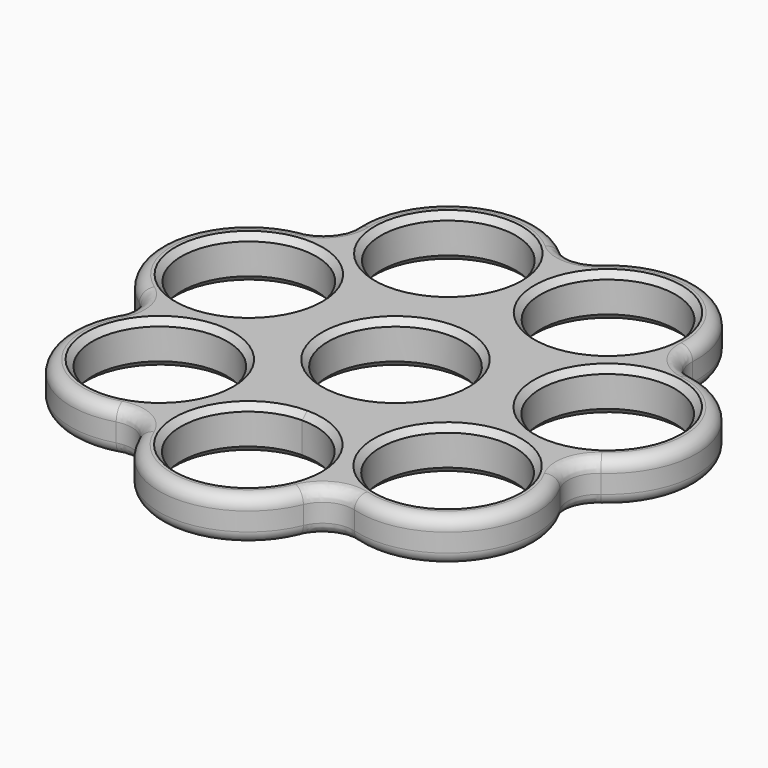
from build123d import *

# Parameters (mm, degrees)
F1_DEPTH = 7
F3_COUNT = 7
F5_R     = 11
F6_DEPTH = 7.001
F7_R     = 5
F8_R     = 2
F9_SIZE  = 1


# Not quite as in the source:
# - a feature names something its author has since deleted; it is built from what else it names


with BuildPart() as f1:
    # F0 (on Top) → F1 (new body)
    with BuildSketch(Plane.XY):
        with BuildLine():
            ThreePointArc((-14.5, 0), (0, -14.5), (14.5, 0))
            ThreePointArc((14.5, 0), (0, 14.5), (-14.5, 0))
        make_face()
        with BuildLine():
            Line((14.5, -30), (14.5, 0))
            ThreePointArc((14.5, 0), (0, -14.5), (-14.5, 0))
            Line((-14.5, 0), (-14.5, -30))
            ThreePointArc((-14.5, -30), (0, -15.5), (14.5, -30))
        make_face()
        with BuildLine():
            ThreePointArc((-14.5, -30), (0, -44.5), (14.5, -30))
            ThreePointArc((14.5, -30), (0, -15.5), (-14.5, -30))
        make_face()
    extrude(amount=F1_DEPTH)


with BuildPart() as f3_1:
    # F3: instance of F1
    add(f1.part.rotate(Axis((0, 0, 13.2415927947), (0, 0, 1)), 1 * 360 / F3_COUNT))


with BuildPart() as f3_2:
    # F3: instance of F1
    add(f1.part.rotate(Axis((0, 0, 13.2415927947), (0, 0, 1)), 2 * 360 / F3_COUNT))


with BuildPart() as f3_3:
    # F3: instance of F1
    add(f1.part.rotate(Axis((0, 0, 13.2415927947), (0, 0, 1)), 3 * 360 / F3_COUNT))


with BuildPart() as f3_4:
    # F3: instance of F1
    add(f1.part.rotate(Axis((0, 0, 13.2415927947), (0, 0, 1)), 4 * 360 / F3_COUNT))


with BuildPart() as f3_5:
    # F3: instance of F1
    add(f1.part.rotate(Axis((0, 0, 13.2415927947), (0, 0, 1)), 5 * 360 / F3_COUNT))


with BuildPart() as f3_6:
    # F3: instance of F1
    add(f1.part.rotate(Axis((0, 0, 13.2415927947), (0, 0, 1)), 6 * 360 / F3_COUNT))


with BuildPart() as f3_5_1:
    add(f3_5.part)

    # F4: union F3_6, F1, F3_1, F3_2, F3_3, F3_4
    add(f3_6.part)
    add(f1.part)
    add(f3_1.part)
    add(f3_2.part)
    add(f3_3.part)
    add(f3_4.part)

    # F5 (on face) → F6 (cut, through all)
    with BuildSketch(Plane.XY.offset(7)):
        with BuildLine():
            ThreePointArc((0, -11), (7.7781745931, -7.7781745931), (11, 0))
            ThreePointArc((11, 0), (-7.7781745931, 7.7781745931), (0, -11))
        make_face()
        with BuildLine():
            ThreePointArc((11, -30), (7.7781745931, -22.2218254069), (0, -19))
            ThreePointArc((0, -19), (-7.7781745931, -37.7781745931), (11, -30))
        make_face()
        with Locations((23.454944474, -18.7046940558)):
            Circle(F5_R)
        with Locations((29.2478373655, 6.6756280187)):
            Circle(F5_R)
        with Locations((13.0165121735, 27.0290660371)):
            Circle(F5_R)
        with Locations((-13.0165121735, 27.0290660371)):
            Circle(F5_R)
        with Locations((-29.2478373655, 6.6756280187)):
            Circle(F5_R)
        with Locations((-23.454944474, -18.7046940558)):
            Circle(F5_R)
    extrude(amount=-F6_DEPTH, mode=Mode.SUBTRACT)

    # F7
    f7_edges = [f3_5_1.edges().sort_by_distance(p)[0] for p in [
        (-26.127363, 20.835877, 3.5),
        (-32.580289, -7.436238, 3.5),
        (-14.499592, -30.108714, 3.5),
        (14.499592, -30.108714, 3.5),
        (32.580289, -7.436238, 3.5),
        (26.127363, 20.835877, 3.5),
        (0, 33.418151, 3.5),
    ]]
    fillet(f7_edges, radius=F7_R)

    # F8
    f8_edges = [f3_5_1.edges().sort_by_distance(p)[0] for p in [
        (34.791501, -27.745296, 7),
        (0, -44.5, 0),
    ]]
    fillet(f8_edges, radius=F8_R)

    # F9
    f9_edges = [f3_5_1.edges().sort_by_distance(p)[0] for p in [
        (0, 11, 7),
        (0, -41, 7),
        (0, -41, 0),
        (0, 11, 0),
        (-34.454944, -18.704694, 7),
        (-40.247837, 6.675628, 7),
        (-24.016512, 27.029066, 7),
        (2.016512, 27.029066, 7),
        (18.247837, 6.675628, 7),
        (12.454944, -18.704694, 7),
        (18.247837, 6.675628, 0),
        (12.454944, -18.704694, 0),
        (-34.454944, -18.704694, 0),
        (-40.247837, 6.675628, 0),
        (-24.016512, 27.029066, 0),
        (2.016512, 27.029066, 0),
    ]]
    chamfer(f9_edges, length=F9_SIZE)


solid = f3_5_1.part
